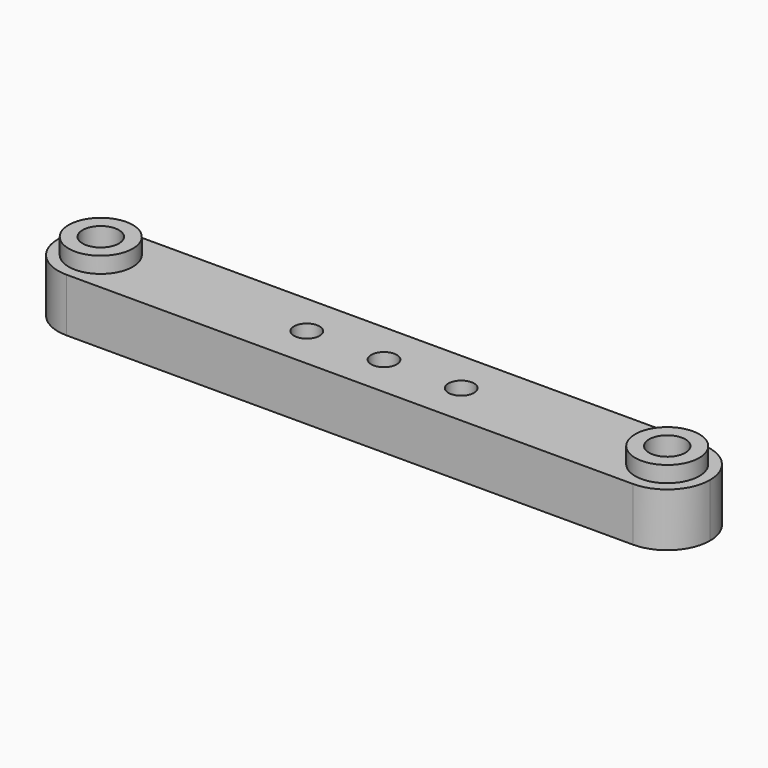
from build123d import *

# Parameters (mm, degrees)
F2_W      = 61
F2_H      = 8
F2_R      = 3
F5_DEPTH  = 5
F1_R      = 3
F1_R_2    = 1.7
F6_DEPTH  = 6.5
F0_R      = 1.7
F7_DEPTH  = 12.5
F3_R      = 2.05
F8_DEPTH  = 2
F9_DEPTH  = 2
F10_R     = 3.99999
F4_R      = 1.2
F11_DEPTH = 6.501


# Not quite as in the source:
# - a fillet or chamfer is up to 0.001 mm smaller than in the source, because OpenCascade refuses the exact size


with BuildPart() as f5:
    # F2 (on face) → F5 (new body)
    with BuildSketch(Plane.XY):
        with Locations((0, 38)):
            Rectangle(F2_W, F2_H)
        with Locations((-26.5, 38)):
            Circle(F2_R, mode=Mode.SUBTRACT)
        Polygon((1.1402667816, 36.025), (0, 36.025), (-1.1402667816, 36.025), (-2.2805335633, 38), (-1.1402667816, 39.975), (0, 39.975), (1.1402667816, 39.975), (2.2805335633, 38), align=None, mode=Mode.SUBTRACT)
        with Locations((26.5, 38)):
            Circle(F2_R, mode=Mode.SUBTRACT)
        Polygon((-1.1402667816, 36.025), (0, 36.025), (1.1402667816, 36.025), (2.2805335633, 38), (1.1402667816, 39.975), (0, 39.975), (-1.1402667816, 39.975), (-2.2805335633, 38), align=None)
        with Locations((-26.5, 38)):
            Circle(F2_R)
        with Locations((26.5, 38)):
            Circle(F2_R)
    extrude(amount=F5_DEPTH)

    # F1 (on Top) → F6 (join)
    with BuildSketch(Plane.XY):
        with Locations((-26.5, 38)):
            Circle(F1_R)
        with Locations((-26.5, 38)):
            Circle(F1_R_2, mode=Mode.SUBTRACT)
        with Locations((26.5, 38)):
            Circle(F1_R)
        with Locations((26.5, 38)):
            Circle(F1_R_2, mode=Mode.SUBTRACT)
    extrude(amount=F6_DEPTH)

    # F0 (on Top) → F7 (cut, symmetric)
    with BuildSketch(Plane.XY):
        with Locations((-26.5, 38)):
            Circle(F0_R)
        with Locations((26.5, 38)):
            Circle(F0_R)
        with Locations((-26.5, -38)):
            Circle(F0_R)
        with Locations((26.5, -38)):
            Circle(F0_R)
    extrude(amount=F7_DEPTH, both=True, mode=Mode.SUBTRACT)

    # F3 (on face) → F8 (cut)
    with BuildSketch(Plane.XY):
        with Locations((-7.225, 38)):
            Circle(F3_R)
        with Locations((7.225, 38)):
            Circle(F3_R)
    extrude(amount=F8_DEPTH, mode=Mode.SUBTRACT)

    # F2 (on face) → F9 (cut)
    with BuildSketch(Plane.XY):
        Polygon((-1.1402667816, 36.025), (0, 36.025), (1.1402667816, 36.025), (2.2805335633, 38), (1.1402667816, 39.975), (0, 39.975), (-1.1402667816, 39.975), (-2.2805335633, 38), align=None)
    extrude(amount=F9_DEPTH, mode=Mode.SUBTRACT)

    # F10 (radius 4 in the source; OpenCascade refuses exactly that, so slightly less here)
    f10_edges = [f5.edges().sort_by_distance(p)[0] for p in [
        (-30.5, 42, 2.5),
        (-30.5, 34, 2.5),
        (30.5, 42, 2.5),
        (30.5, 34, 2.5),
    ]]
    fillet(f10_edges, radius=F10_R)

    # F4 (on face) → F11 (cut, through all)
    with BuildSketch(Plane.XY):
        with Locations((-7.225, 38)):
            Circle(F4_R)
        with Locations((0, 38)):
            Circle(F4_R)
        with Locations((7.225, 38)):
            Circle(F4_R)
    extrude(amount=F11_DEPTH, mode=Mode.SUBTRACT)


solid = f5.part
